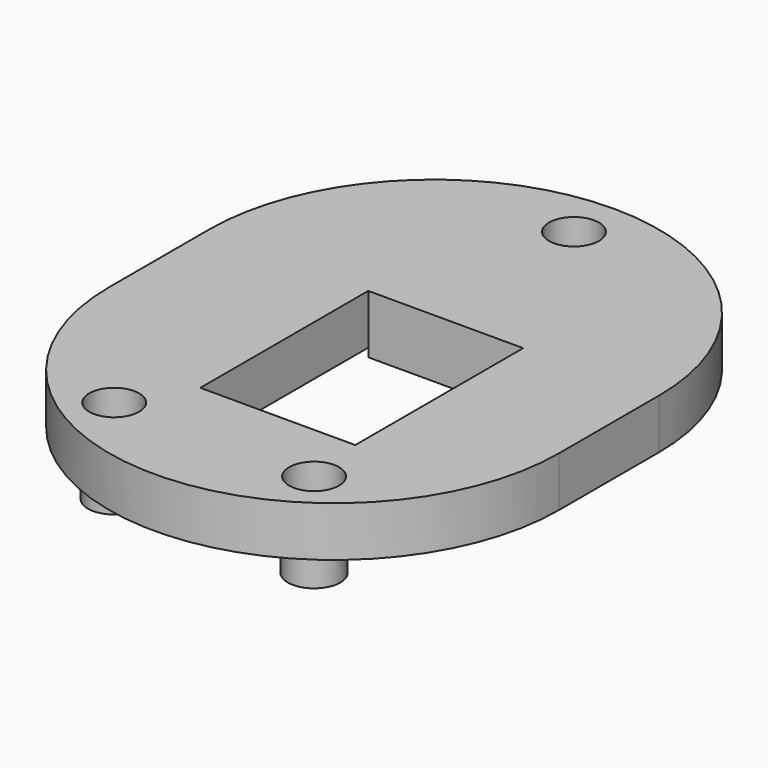
from build123d import *

# Parameters (mm, degrees)
F1_DEPTH    = 10
F3_R        = 44.99999
F4_W        = 31
F4_H        = 42
F5_DEPTH    = 11
F6_R        = 5.25
F7_DEPTH    = 7
F9_D        = 10
F9_DEPTH    = 10.001
F10_D       = 6.5
F10_ON_F6_D = 6.5
F11_W       = 31
F11_H       = 2.5
F12_DEPTH   = 1.7
F13_W       = 2.5
F13_H       = 14.5
F14_DEPTH   = 1.7
F16_DEPTH   = 25


# Not quite as in the source:
# - a fillet or chamfer is up to 0.001 mm smaller than in the source, because OpenCascade refuses the exact size


with BuildPart() as f1:
    # F0 (on Top) → F1 (new body)
    with BuildSketch(Plane.XY):
        with BuildLine():
            Line((-45, 70), (-45, 0))
            ThreePointArc((-45, 0), (0, -45), (45, 0))
            Line((45, 0), (45, 70))
            Line((45, 70), (-45, 70))
        make_face()
    extrude(amount=F1_DEPTH)

    # F3 (radius 45 in the source; OpenCascade refuses exactly that, so slightly less here)
    f3_edges = [f1.edges().sort_by_distance(p)[0] for p in [
        (-45, 70, 5),
        (45, 70, 5),
    ]]
    fillet(f3_edges, radius=F3_R)

    # F4 (on face) → F5 (cut)
    with BuildSketch(Plane.XY.offset(10)):
        with Locations((2.9, 3.3)):
            Rectangle(F4_W, F4_H)
    extrude(amount=-F5_DEPTH, mode=Mode.SUBTRACT)

    # F6 (on face) → F7 (join)
    with BuildSketch(Plane(origin=(0, 0, 0), x_dir=(1, 0, 0), z_dir=(0, 0, -1))):
        with Locations((0, -60)):
            Circle(F6_R)
        with Locations((-20, 30)):
            Circle(F6_R)
        with Locations((20, 30)):
            Circle(F6_R)
    extrude(amount=F7_DEPTH)

    # F9 (through all, one way)
    with BuildSketch(Plane(origin=(0, 0, 0), x_dir=(1, 0, 0), z_dir=(0, 0, -1))):
        with Locations((-20, 30), (20, 30), (0, -60)):
            Circle(F9_D / 2)
    extrude(amount=-F9_DEPTH, mode=Mode.SUBTRACT)

    # F10 (through all)
    with Locations(Plane.XY):
        with Locations((20, -30), (0, 60)):
            Hole(F10_D / 2)

    # F10 on F6 (through all)
    with Locations(Plane.XY):
        with Locations((-20, -30)):
            Hole(F10_ON_F6_D / 2)

    # F11 (on face) → F12 (join)
    with BuildSketch(Plane(origin=(0, 0, 0), x_dir=(1, 0, 0), z_dir=(0, 0, -1))):
        with Locations((2.9, -25.55)):
            Rectangle(F11_W, F11_H)
    extrude(amount=F12_DEPTH)

    # F13 (on face) → F14 (join)
    with BuildSketch(Plane(origin=(0, 0, 0), x_dir=(1, 0, 0), z_dir=(0, 0, -1))):
        with Locations((-38.25, 6.55)):
            Rectangle(F13_W, F13_H)
    extrude(amount=F14_DEPTH)

    # F15 (on face) → F16 (cut)
    with BuildSketch(Plane(origin=(-39.5, 0, 0), x_dir=(0, -1, 0), z_dir=(-1, 0, 0))):
        Polygon((13, -1), (13, 0), (0, 0), (0, -1), (2.55, -1), (2.55, -1.7), (10.55, -1.7), (10.55, -1), align=None)
    extrude(amount=-F16_DEPTH, mode=Mode.SUBTRACT)


solid = f1.part
